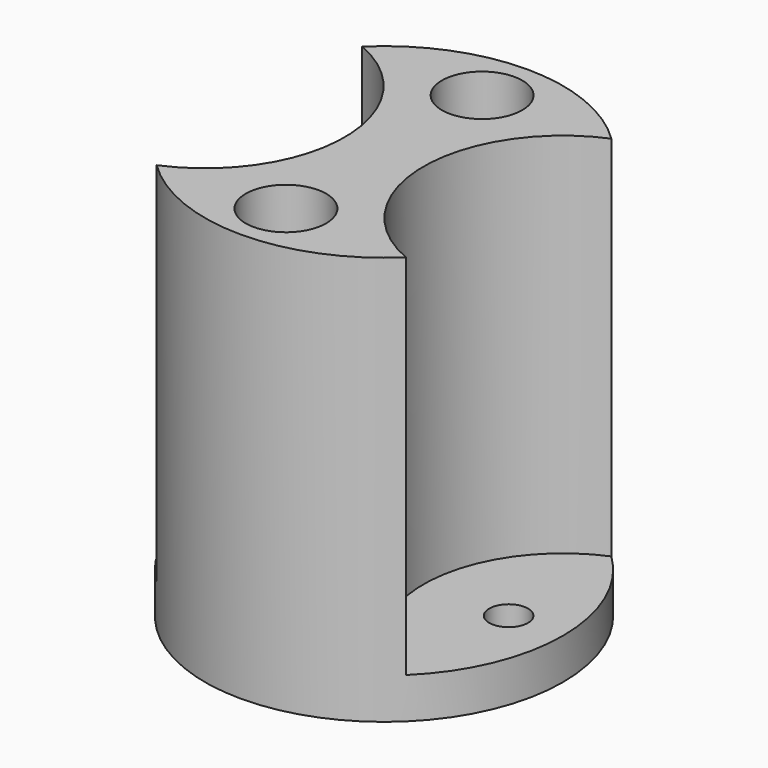
from build123d import *
from build123d import SkipClean  # not in build123d's __all__

# Parameters (mm, degrees)
F0_R     = 1.2065
F1_DEPTH = 2.54
F3_DEPTH = 22.86
F4_R     = 2.5
F5_DEPTH = 6.35


# Not quite as in the source:
# - a feature names something its author has since deleted; it is built from what else it names


with BuildPart() as f1:
    # F0 (on Top) → F1 (new body)
    with BuildSketch(Plane.XY):
        with BuildLine():
            ThreePointArc((7.747, -7.9846143326), (2.4553498698, 0), (7.747, 7.9846143326))
            ThreePointArc((7.747, 7.9846143326), (0, 11.1252), (-7.747, 7.9846143326))
            ThreePointArc((-7.747, 7.9846143326), (-2.4553498698, 0), (-7.747, -7.9846143326))
            ThreePointArc((-7.747, -7.9846143326), (0, -11.1252), (7.747, -7.9846143326))
        make_face()
        with BuildLine():
            ThreePointArc((-7.747, -7.9846143326), (-2.4553498698, 0), (-7.747, 7.9846143326))
            ThreePointArc((-7.747, 7.9846143326), (-11.1252, 0), (-7.747, -7.9846143326))
        make_face()
        with Locations((-7.747, 0)):
            Circle(F0_R, mode=Mode.SUBTRACT)
        with BuildLine():
            ThreePointArc((7.747, -7.9846143326), (10.245901606, -4.3349250651), (11.1252, 0))
            ThreePointArc((11.1252, 0), (10.245901606, 4.3349250651), (7.747, 7.9846143326))
            ThreePointArc((7.747, 7.9846143326), (2.4553498698, 0), (7.747, -7.9846143326))
        make_face()
        with Locations((7.747, 0)):
            Circle(F0_R, mode=Mode.SUBTRACT)
    extrude(amount=F1_DEPTH)

    # F2 (on face) → F3 (join)
    with BuildSketch(Plane.XY.offset(2.54)):
        with BuildLine():
            ThreePointArc((-7.747, 7.9846143326), (-2.4553498698, 0), (-7.747, -7.9846143326))
            ThreePointArc((-7.747, -7.9846143326), (0, -11.1252), (7.747, -7.9846143326))
            ThreePointArc((7.747, -7.9846143326), (2.4553498698, 0), (7.747, 7.9846143326))
            ThreePointArc((7.747, 7.9846143326), (0, 11.1252), (-7.747, 7.9846143326))
        make_face()
    with SkipClean():  # cleaning this boolean's faces spoils the solid; the shape is the same uncleaned
        extrude(amount=F3_DEPTH)

    # F4 (on face) → F5 (cut)
    with BuildSketch(Plane.XY.offset(25.4)):
        with Locations((0, 7.62)):
            Circle(F4_R)
        with Locations((0, -7.62)):
            Circle(F4_R)
    extrude(amount=-F5_DEPTH, mode=Mode.SUBTRACT)


solid = f1.part
